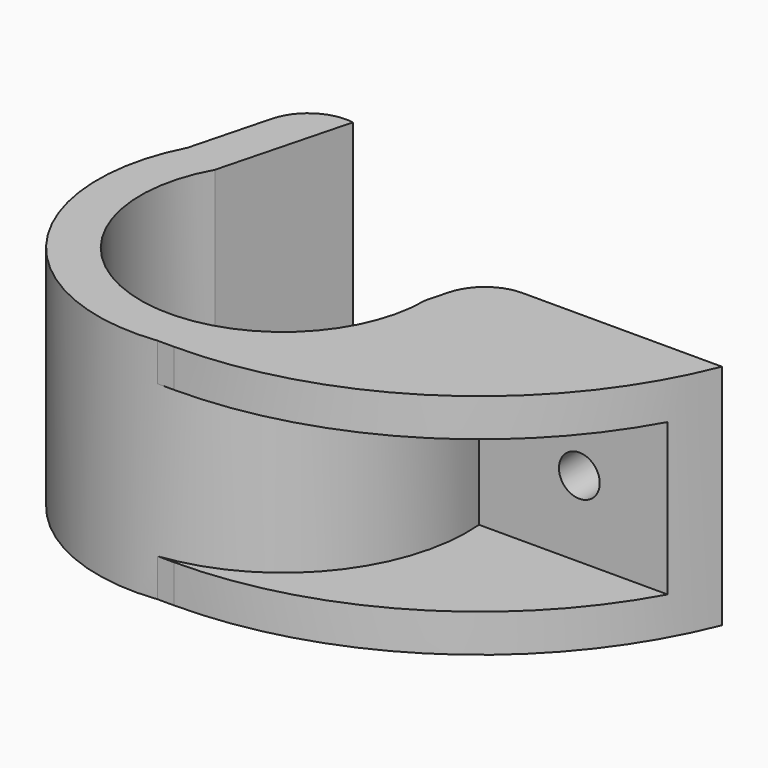
from build123d import *

# Parameters (mm, degrees)
F1_DEPTH    = 24
F3_W        = 41.439505011
F3_H        = 4
F4_DEPTH    = 25
F5_DEPTH    = 25
F6_DEPTH    = 25
F7_T1_DEPTH = 191.2806862556
F7_T3_DEPTH = 191.2806862556
F8_R        = 5
F9_T1_DEPTH = 48.8746859277
F11_D       = 4.3


# Not quite as in the source:
# - a fillet or chamfer that OpenCascade refuses, or shapes differently, is made with other operations: its cross-section is extruded or revolved along the edge and cut away or added


with BuildPart() as f1:
    # F0 (on Top) → F1 (new body)
    with BuildSketch(Plane.XY):
        with BuildLine():
            ThreePointArc((15, 0), (-3.8035773729, -14.5097484185), (-13.0710398891, 7.3585267695))
            Line((-13.0710398891, 7.3585267695), (-9.4777092406, 21.0662336417))
            Line((-9.4777092406, 21.0662336417), (-13.8306337662, 22.2073068536))
            Line((-13.8306337662, 22.2073068536), (-17.2866620502, 9.0233760402))
            ThreePointArc((-17.2866620502, 9.0233760402), (-3.8959382238, -19.1068486506), (19.439505011, 1.5348110402))
            Line((19.439505011, 1.5348110402), (41.439505011, 1.5348110402))
            Line((41.439505011, 1.5348110402), (41.439505011, 6.0348110402))
            Line((41.439505011, 6.0348110402), (16.5819620065, 6.0348110402))
            Line((16.5819620065, 6.0348110402), (15, 0))
        make_face()
    extrude(amount=F1_DEPTH)

    # F3 (on offset) → F4 (join)
    with BuildSketch(Plane.XZ.offset(19.3651889598)):
        with Locations((20.7197525055, 2)):
            Rectangle(F3_W, F3_H)
        with Locations((20.7197525055, 22)):
            Rectangle(F3_W, F3_H)
    extrude(amount=-F4_DEPTH)

    # F5 (cut): a face of the model
    f5_faces = [f1.faces().sort_by_distance(p)[0] for p in [
        (6.8703868354, -3.2827389678, 20),
    ]]
    extrude(f5_faces, amount=-F5_DEPTH, mode=Mode.SUBTRACT)

    # F6 (cut): a face of the model
    f6_faces = [f1.faces().sort_by_distance(p)[0] for p in [
        (6.8703868354, -3.2827389678, 4),
    ]]
    extrude(f6_faces, amount=-F6_DEPTH, mode=Mode.SUBTRACT)

    # F7: fillet of radius 40.3173664916 on 2 edges, made by hand

    # F7_s2 → F7_t1 (cut)
    with BuildSketch(Plane.XY.offset(-73.6403431278)):
        with BuildLine():
            ThreePointArc((3.9833677598, -19.3651889598), (26.6114599119, -12.4163628374), (41.439505011, 6.0348110402))
            Line((41.439505011, 6.0348110402), (42.188627756, 5.7364637104))
            ThreePointArc((42.188627756, 5.7364637104), (42.2458523408, -6.6651889598), (42.2458523408, -19.3651889598))
            Line((42.2458523408, -19.3651889598), (41.439505011, -20.1715362896))
            Line((41.439505011, -20.1715362896), (3.9833677598, -20.1715362896))
            Line((3.9833677598, -20.1715362896), (3.9833677598, -19.3651889598))
        make_face()
    extrude(amount=F7_T1_DEPTH, mode=Mode.SUBTRACT)

    # F7_s4 → F7_t3 (cut)
    with BuildSketch(Plane.XY.offset(-93.6403431278)):
        with BuildLine():
            ThreePointArc((3.9833677598, -19.3651889598), (26.6114599119, -12.4163628374), (41.439505011, 6.0348110402))
            Line((41.439505011, 6.0348110402), (42.188627756, 5.7364637104))
            ThreePointArc((42.188627756, 5.7364637104), (42.2458523408, -6.6651889598), (42.2458523408, -19.3651889598))
            Line((42.2458523408, -19.3651889598), (41.439505011, -20.1715362896))
            Line((41.439505011, -20.1715362896), (3.9833677598, -20.1715362896))
            Line((3.9833677598, -20.1715362896), (3.9833677598, -19.3651889598))
        make_face()
    extrude(amount=F7_T3_DEPTH, mode=Mode.SUBTRACT)

    # F8
    f8_edges = [f1.edges().sort_by_distance(p)[0] for p in [
        (16.581962, 6.034811, 12),
    ]]
    fillet(f8_edges, radius=F8_R)

    # F9: fillet of radius 5 on 1 edges, made by hand

    # F9_s2 → F9_t1 (cut)
    with BuildSketch(Plane.XY.offset(-12.4373429638)):
        with BuildLine():
            ThreePointArc((-9.4777092406, 21.0662336417), (-12.9919549133, 20.3118564706), (-15.0921376669, 17.394967723))
            Line((-15.0921376669, 17.394967723), (-13.8306337662, 22.2073068536))
            Line((-13.8306337662, 22.2073068536), (-9.4777092406, 21.0662336417))
        make_face()
    extrude(amount=F9_T1_DEPTH, mode=Mode.SUBTRACT)

    # F11 (through all)
    with Locations(Plane.XZ.offset(-1.5348110402)):
        with Locations((30.0100483, 12)):
            Hole(F11_D / 2)


solid = f1.part
